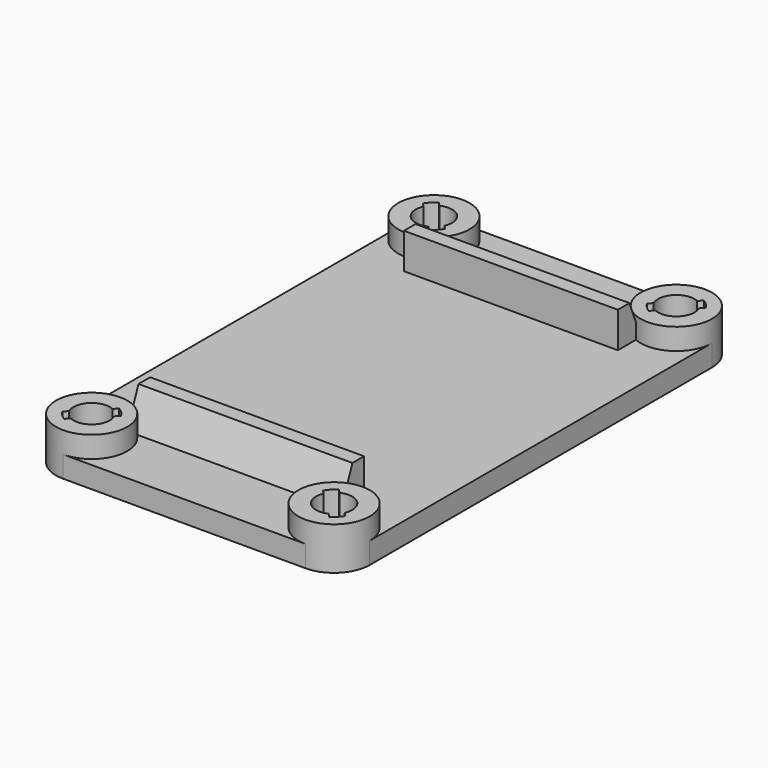
from build123d import *

# Parameters (mm, degrees)
F1_DEPTH    = 3
F3_DEPTH    = 6
F5_DEPTH    = 12.5
F6_W        = 30
F6_H        = 2.0356480181
F7_DEPTH    = 8
F8_T4_DEPTH = 30
F8_T9_DEPTH = 30


# Not quite as in the source:
# - a fillet or chamfer that OpenCascade refuses, or shapes differently, is made with other operations: its cross-section is extruded or revolved along the edge and cut away or added


with BuildPart() as f1:
    # F0 (on Top) → F1 (new body)
    with BuildSketch(Plane.XY):
        with BuildLine():
            ThreePointArc((22, 30), (20.5355339059, 33.5355339059), (17, 35))
            Line((17, 35), (-17, 35))
            ThreePointArc((-17, 35), (-20.5355339059, 33.5355339059), (-22, 30))
            Line((-22, 30), (-22, -30))
            ThreePointArc((-22, -30), (-20.5355339059, -33.5355339059), (-17, -35))
            Line((-17, -35), (17, -35))
            ThreePointArc((17, -35), (20.5355339059, -33.5355339059), (22, -30))
            Line((22, -30), (22, 30))
        make_face()
    extrude(amount=F1_DEPTH)

    # F2 (on Top) → F3 (join)
    with BuildSketch(Plane.XY):
        with BuildLine():
            ThreePointArc((-12, 30), (-13.4644661049, 33.5355339167), (-17.0000000305, 35))
            ThreePointArc((-17.0000000305, 35), (-20.5355339275, 33.5355338843), (-22, 29.9999999695))
            ThreePointArc((-22, 29.9999999695), (-16.9999999847, 25), (-12, 30))
        make_face()
        with BuildLine():
            ThreePointArc((22, 30), (20.5355339059, 33.5355339059), (17, 35))
            ThreePointArc((17, 35), (13.4644660941, 26.4644660941), (22, 30))
        make_face()
        with BuildLine():
            ThreePointArc((17, -35), (20.5355339059, -33.5355339059), (22, -30))
            ThreePointArc((22, -30), (13.4644660941, -26.4644660941), (17, -35))
        make_face()
        with BuildLine():
            ThreePointArc((-12, -30), (-17, -25), (-22, -30))
            ThreePointArc((-22, -30), (-20.5355339059, -33.5355339059), (-17, -35))
            ThreePointArc((-17, -35), (-13.4644660941, -33.5355339059), (-12, -30))
        make_face()
    extrude(amount=F3_DEPTH)

    # F4 (on Top) → F5 (cut, symmetric)
    with BuildSketch(Plane.XY):
        with BuildLine():
            ThreePointArc((-18.0685374254, -32.3153245497), (-15.6256402281, -32.1479374333), (-14.45, -30))
            ThreePointArc((-14.45, -30), (-14.5093597608, -29.4529979899), (-14.6846754503, -28.9314625746))
            Line((-14.6846754503, -28.9314625746), (-18.0685374254, -32.3153245497))
        make_face()
        with BuildLine():
            Line((-18.0685374254, -32.3153245497), (-14.6846754503, -28.9314625746))
            ThreePointArc((-14.6846754503, -28.9314625746), (-15.196877708, -28.196877708), (-15.9314625746, -27.6846754503))
            Line((-15.9314625746, -27.6846754503), (-19.3153245497, -31.0685374254))
            ThreePointArc((-19.3153245497, -31.0685374254), (-18.803122292, -31.803122292), (-18.0685374254, -32.3153245497))
        make_face()
        with BuildLine():
            ThreePointArc((-15.9314625746, -27.6846754503), (-15.196877708, -28.196877708), (-14.6846754503, -28.9314625746))
            Line((-14.6846754503, -28.9314625746), (-14.16467731, -28.4114644343))
            ThreePointArc((-14.16467731, -28.4114644343), (-14.7019029611, -27.7019029611), (-15.4114644343, -27.16467731))
            Line((-15.4114644343, -27.16467731), (-15.9314625746, -27.6846754503))
        make_face()
        with BuildLine():
            Line((-18.5885355657, -32.83532269), (-18.0685374254, -32.3153245497))
            ThreePointArc((-18.0685374254, -32.3153245497), (-18.803122292, -31.803122292), (-19.3153245497, -31.0685374254))
            Line((-19.3153245497, -31.0685374254), (-19.83532269, -31.5885355657))
            ThreePointArc((-19.83532269, -31.5885355657), (-19.2980970389, -32.2980970389), (-18.5885355657, -32.83532269))
        make_face()
        with BuildLine():
            Line((-19.3153245497, -31.0685374254), (-15.9314625746, -27.6846754503))
            ThreePointArc((-15.9314625746, -27.6846754503), (-18.803122292, -28.196877708), (-19.3153245497, -31.0685374254))
        make_face()
        with BuildLine():
            ThreePointArc((19.3153245497, -31.0685374254), (19.4906402392, -30.5470020101), (19.55, -30))
            ThreePointArc((19.55, -30), (18.3743597719, -27.8520625667), (15.9314625746, -27.6846754503))
            Line((15.9314625746, -27.6846754503), (19.3153245497, -31.0685374254))
        make_face()
        with BuildLine():
            Line((19.3153245497, -31.0685374254), (15.9314625746, -27.6846754503))
            ThreePointArc((15.9314625746, -27.6846754503), (15.196877708, -28.196877708), (14.6846754503, -28.9314625746))
            Line((14.6846754503, -28.9314625746), (18.0685374254, -32.3153245497))
            ThreePointArc((18.0685374254, -32.3153245497), (18.803122292, -31.803122292), (19.3153245497, -31.0685374254))
        make_face()
        with BuildLine():
            ThreePointArc((14.6846754503, -28.9314625746), (15.196877708, -28.196877708), (15.9314625746, -27.6846754503))
            Line((15.9314625746, -27.6846754503), (15.4114644343, -27.16467731))
            ThreePointArc((15.4114644343, -27.16467731), (14.7019029611, -27.7019029611), (14.16467731, -28.4114644343))
            Line((14.16467731, -28.4114644343), (14.6846754503, -28.9314625746))
        make_face()
        with BuildLine():
            Line((19.83532269, -31.5885355657), (19.3153245497, -31.0685374254))
            ThreePointArc((19.3153245497, -31.0685374254), (18.803122292, -31.803122292), (18.0685374254, -32.3153245497))
            Line((18.0685374254, -32.3153245497), (18.5885355657, -32.83532269))
            ThreePointArc((18.5885355657, -32.83532269), (19.2980970389, -32.2980970389), (19.83532269, -31.5885355657))
        make_face()
        with BuildLine():
            Line((18.0685374254, -32.3153245497), (14.6846754503, -28.9314625746))
            ThreePointArc((14.6846754503, -28.9314625746), (15.196877708, -31.803122292), (18.0685374254, -32.3153245497))
        make_face()
        with BuildLine():
            ThreePointArc((15.9314625746, 27.6846754503), (18.3743597719, 27.8520625667), (19.55, 30))
            ThreePointArc((19.55, 30), (19.4906402392, 30.5470020101), (19.3153245497, 31.0685374254))
            Line((19.3153245497, 31.0685374254), (15.9314625746, 27.6846754503))
        make_face()
        with BuildLine():
            Line((15.9314625746, 27.6846754503), (19.3153245497, 31.0685374254))
            ThreePointArc((19.3153245497, 31.0685374254), (18.803122292, 31.803122292), (18.0685374254, 32.3153245497))
            Line((18.0685374254, 32.3153245497), (14.6846754503, 28.9314625746))
            ThreePointArc((14.6846754503, 28.9314625746), (15.196877708, 28.196877708), (15.9314625746, 27.6846754503))
        make_face()
        with BuildLine():
            ThreePointArc((18.0685374254, 32.3153245497), (18.803122292, 31.803122292), (19.3153245497, 31.0685374254))
            Line((19.3153245497, 31.0685374254), (19.83532269, 31.5885355657))
            ThreePointArc((19.83532269, 31.5885355657), (19.2980970389, 32.2980970389), (18.5885355657, 32.83532269))
            Line((18.5885355657, 32.83532269), (18.0685374254, 32.3153245497))
        make_face()
        with BuildLine():
            Line((15.4114644343, 27.16467731), (15.9314625746, 27.6846754503))
            ThreePointArc((15.9314625746, 27.6846754503), (15.196877708, 28.196877708), (14.6846754503, 28.9314625746))
            Line((14.6846754503, 28.9314625746), (14.16467731, 28.4114644343))
            ThreePointArc((14.16467731, 28.4114644343), (14.7019029611, 27.7019029611), (15.4114644343, 27.16467731))
        make_face()
        with BuildLine():
            Line((14.6846754503, 28.9314625746), (18.0685374254, 32.3153245497))
            ThreePointArc((18.0685374254, 32.3153245497), (15.196877708, 31.803122292), (14.6846754503, 28.9314625746))
        make_face()
        with BuildLine():
            ThreePointArc((-14.6846754503, 28.9314625746), (-14.5093597608, 29.4529979899), (-14.45, 30))
            ThreePointArc((-14.45, 30), (-15.6256402281, 32.1479374333), (-18.0685374254, 32.3153245497))
            Line((-18.0685374254, 32.3153245497), (-14.6846754503, 28.9314625746))
        make_face()
        with BuildLine():
            Line((-14.6846754503, 28.9314625746), (-18.0685374254, 32.3153245497))
            ThreePointArc((-18.0685374254, 32.3153245497), (-18.803122292, 31.803122292), (-19.3153245497, 31.0685374254))
            Line((-19.3153245497, 31.0685374254), (-15.9314625746, 27.6846754503))
            ThreePointArc((-15.9314625746, 27.6846754503), (-15.196877708, 28.196877708), (-14.6846754503, 28.9314625746))
        make_face()
        with BuildLine():
            ThreePointArc((-19.3153245497, 31.0685374254), (-18.803122292, 31.803122292), (-18.0685374254, 32.3153245497))
            Line((-18.0685374254, 32.3153245497), (-18.5885355657, 32.83532269))
            ThreePointArc((-18.5885355657, 32.83532269), (-19.2980970389, 32.2980970389), (-19.83532269, 31.5885355657))
            Line((-19.83532269, 31.5885355657), (-19.3153245497, 31.0685374254))
        make_face()
        with BuildLine():
            Line((-14.16467731, 28.4114644343), (-14.6846754503, 28.9314625746))
            ThreePointArc((-14.6846754503, 28.9314625746), (-15.196877708, 28.196877708), (-15.9314625746, 27.6846754503))
            Line((-15.9314625746, 27.6846754503), (-15.4114644343, 27.16467731))
            ThreePointArc((-15.4114644343, 27.16467731), (-14.7019029611, 27.7019029611), (-14.16467731, 28.4114644343))
        make_face()
        with BuildLine():
            Line((-15.9314625746, 27.6846754503), (-19.3153245497, 31.0685374254))
            ThreePointArc((-19.3153245497, 31.0685374254), (-18.803122292, 28.196877708), (-15.9314625746, 27.6846754503))
        make_face()
    extrude(amount=F5_DEPTH, both=True, mode=Mode.SUBTRACT)

    # F6 (on Top) → F7 (join)
    with BuildSketch(Plane.XY):
        with Locations((0, 23.2678240091)):
            Rectangle(F6_W, F6_H)
        with Locations((0, -23.2678240091)):
            Rectangle(F6_W, F6_H)
    extrude(amount=F7_DEPTH)

    # F8: chamfer of 5 x 2 on 2 edges, made by hand


with BuildPart() as f8_tool2:
    # F8_s3 → F8_t4 (new body)
    with BuildSketch(Plane.YZ.offset(-15)):
        Polygon((26.2856480181, 3), (24.2856480181, 8), (24.2856480181, 3), align=None)
    extrude(amount=F8_T4_DEPTH)

    split(bisect_by=Plane.XY.offset(8), keep=Keep.BOTTOM)


with BuildPart() as f1_1:
    add(f1.part)

    # F8_t1: union F8_tool2
    add(f8_tool2.part)


with BuildPart() as f8_tool7:
    # F8_s8 → F8_t9 (new body)
    with BuildSketch(Plane.YZ.offset(15)):
        Polygon((-26.2856480181, 3), (-24.2856480181, 8), (-24.2856480181, 3), align=None)
    extrude(amount=-F8_T9_DEPTH)

    split(bisect_by=Plane.XY.offset(8), keep=Keep.BOTTOM)


with BuildPart() as f1_2:
    add(f1_1.part)

    # F8_t6: union F8_tool7
    add(f8_tool7.part)


solid = f1_2.part
